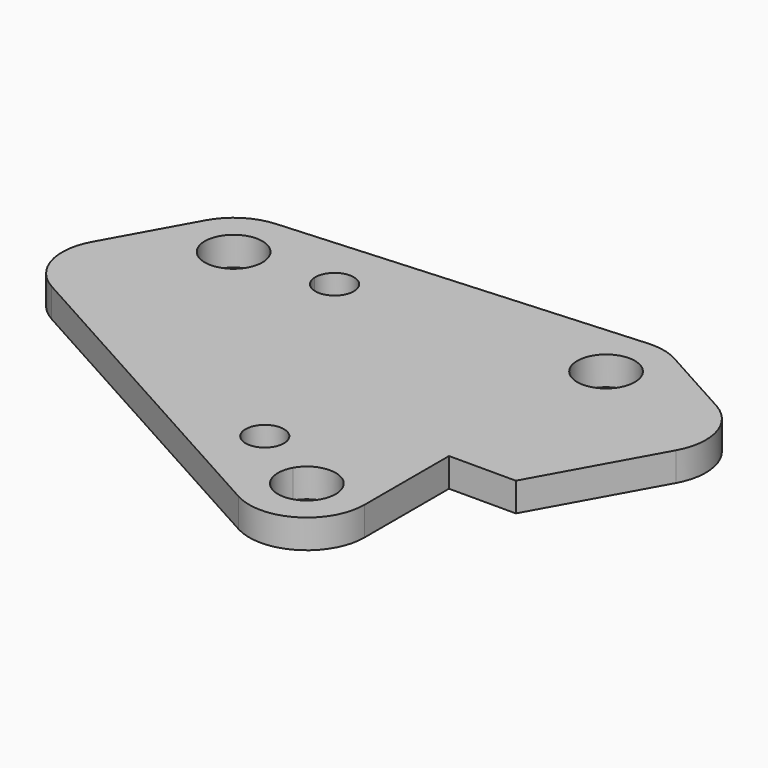
from build123d import *

# Parameters (mm, degrees)
F0_R     = 4.7625
F1_DEPTH = 4.7625


# Not quite as in the source:
# - a length typed as a fraction of an inch, garbled in the dataset ("3 / 203.2 mm" for 3/8 in), is restored


with BuildPart() as f1:
    # F0 (on Top) → F1 (new body)
    with BuildSketch(Plane.XY):
        with BuildLine():
            Line((-60.1561630362, 22.4546581751), (-4.6178116328, -8.3307527105))
            ThreePointArc((-4.6178116328, -8.3307527105), (4.8343029072, -8.2070177532), (9.525, 0))
            Line((9.525, 0), (9.525, 17.4625))
            Line((9.525, 17.4625), (20.5700693075, 17.4625))
            Line((20.5700693075, 17.4625), (31.4198108747, 37.0359519197))
            ThreePointArc((31.4198108747, 37.0359519197), (32.245075818, 44.2792093667), (27.7068697971, 49.984516263))
            Line((27.7068697971, 49.984516263), (15.2107407313, 56.9112337123))
            ThreePointArc((15.2107407313, 56.9112337123), (12.6684281132, 57.8766054007), (9.9569358455, 58.0842243475))
            Line((9.9569358455, 58.0842243475), (-48.4779919349, 54.1737420822))
            ThreePointArc((-48.4779919349, 54.1737420822), (-52.9477518555, 52.7109507654), (-56.1727513924, 49.2878103693))
            Line((-56.1727513924, 49.2878103693), (-63.8691041139, 35.4032225185))
            ThreePointArc((-63.8691041139, 35.4032225185), (-64.6943690572, 28.1599650715), (-60.1561630362, 22.4546581751))
        make_face()
        with BuildLine():
            ThreePointArc((-9.3211290658, 6.9267174493), (-9.4222603076, 6.1317609364), (-9.7192114956, 5.387446905))
            ThreePointArc((-9.7192114956, 5.387446905), (-15.569997824, 7.7216739621), (-9.3211290658, 6.9267174493))
        make_face(mode=Mode.SUBTRACT)
        with BuildLine():
            ThreePointArc((4.7625, 0), (-1.1924347693, -4.6108031373), (-4.1653763553, 2.3089058164))
            ThreePointArc((-4.1653763553, 2.3089058164), (1.1924347693, 4.6108031373), (4.7625, 0))
        make_face(mode=Mode.SUBTRACT)
        with BuildLine():
            ThreePointArc((-43.0794986819, 44.6699987365), (-52.6018408585, 44.510911641), (-43.0901270091, 44.987995363))
            ThreePointArc((-43.0901270091, 44.987995363), (-43.0821565054, 44.829085832), (-43.0794986819, 44.6699987365))
        make_face(mode=Mode.SUBTRACT)
        with BuildLine():
            ThreePointArc((-28.827426439, 45.7299874915), (-31.8963683753, 42.5567593737), (-35.1703408876, 45.5179897405))
            ThreePointArc((-35.1703408876, 45.5179897405), (-32.1084845027, 48.9032156092), (-28.827426439, 45.7299874915))
        make_face(mode=Mode.SUBTRACT)
        with Locations((10.5929290985, 48.5804810018)):
            Circle(F0_R, mode=Mode.SUBTRACT)
    extrude(amount=F1_DEPTH)


solid = f1.part
